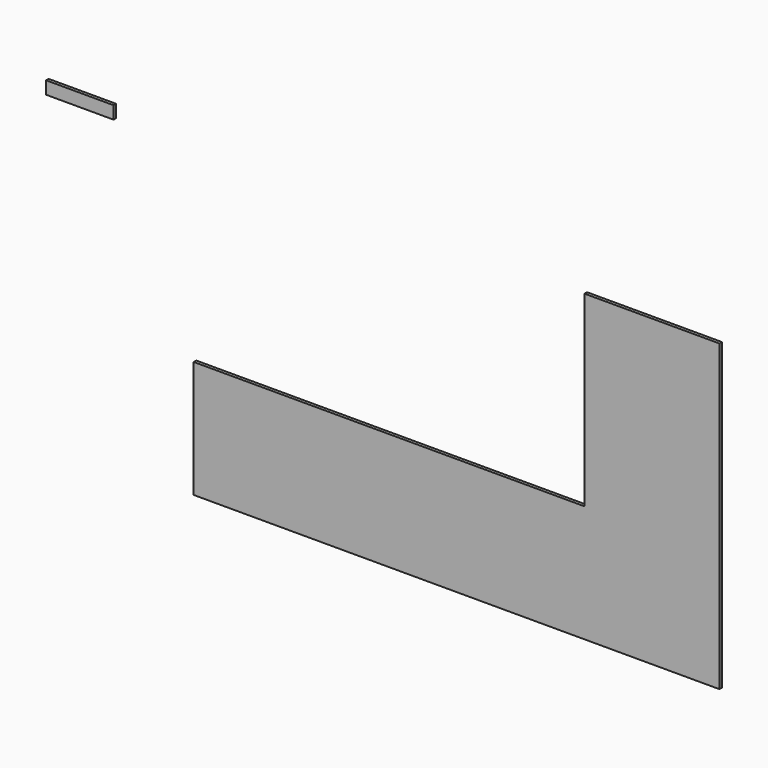
from build123d import *

# Parameters (mm, degrees)
F0_W     = 530
F0_H     = 100
F1_DEPTH = 25
F0_W_2   = 3070
F0_H_2   = 920
F0_W_3   = 543.6974744081
F0_W_4   = 516.3025255919
F0_H_3   = 1471


with BuildPart() as f1:
    # F0 (on Front) → F1 (new body)
    with BuildSketch(Plane.XZ):
        with Locations((-2536.2168025541, 827.7740448676)):
            Rectangle(F0_W, F0_H)
    extrude(amount=-F1_DEPTH)


with BuildPart() as f1b:
    # F0 (on Front) → F1, piece 2 (new body)
    with BuildSketch(Plane.XZ):
        with Locations((-106.2168025541, -1153.2259551324)):
            Rectangle(F0_W_2, F0_H_2)
        with Locations((1700.63193465, -1153.2259551324)):
            Rectangle(F0_W_3, F0_H_2)
        with Locations((2230.63193465, -1153.2259551324)):
            Rectangle(F0_W_4, F0_H_2)
        with Locations((1700.63193465, 42.2740448676)):
            Rectangle(F0_W_3, F0_H_3)
        with Locations((2230.63193465, 42.2740448676)):
            Rectangle(F0_W_4, F0_H_3)
    extrude(amount=-F1_DEPTH)


solid = Compound([f1.part, f1b.part])
